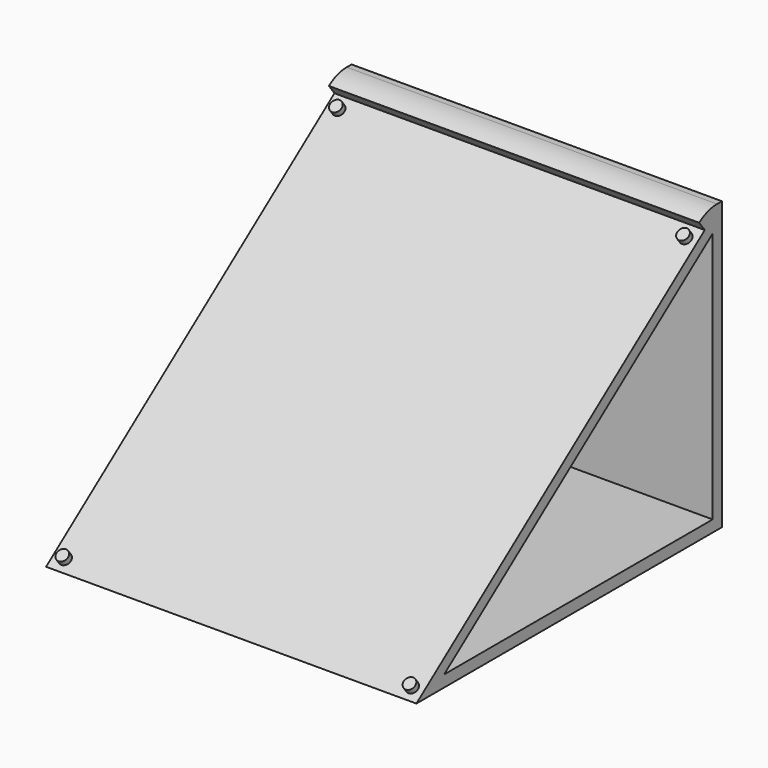
from build123d import *

# Parameters (mm, degrees)
F1_DEPTH  = 50.8
F2_W      = 50.8
F2_H      = 63.5
F2_W_2    = 44.45
F2_H_2    = 57.15
F3_DEPTH  = 1.5875
F5_DEPTH  = 50.8
F6_R      = 5.08
F7_R      = 6.35
F8_DEPTH  = 1.5875
F9_W      = 50.8
F9_H      = 61.8066666667
F9_W_2    = 44.45
F9_H_2    = 57.15
F10_DEPTH = 1.5875
F11_R     = 0.79375
F12_DEPTH = 0.79375
F14_DEPTH = 50.8
F16_DEPTH = 1.5875
F17_T     = -0.79375
F17_2_T   = -0.79375
F17_3_T   = -0.79375
F17_4_T   = -0.79375
F17_5_T   = -0.79375
F17_6_T   = -0.79375
F17_7_T   = -0.79375
F17_8_T   = -0.79375
F17_9_T   = -0.79375
F17_10_T  = -0.79375
F17_11_T  = -0.79375
F17_12_T  = -0.79375
F17_13_T  = -0.79375
F17_14_T  = -0.79375
F17_15_T  = -0.79375
F17_16_T  = -0.79375
F17_17_T  = -0.79375
F17_18_T  = -0.79375
F17_19_T  = -0.79375
F17_20_T  = -0.79375
F17_21_T  = -0.79375
F18_DEPTH = 0.396875


with BuildPart() as f1:
    # F0 (on Right) → F1 (new body)
    with BuildSketch(Plane.YZ):
        Polygon((0, 36.115625), (0, 0), (1.5875, 0), (1.5875, 38.1), (0, 38.1), (-50.8, 0), (-48.1541666667, 0), align=None)
    extrude(amount=F1_DEPTH)

    # F2 (on face) → F3 (join)
    with BuildSketch(Plane(origin=(0, -18.288, 24.384), x_dir=(1, 0, 0), z_dir=(0, -0.6, 0.8))):
        with Locations((25.4, -8.89)):
            Rectangle(F2_W, F2_H)
        with Locations((25.4, -8.89)):
            Rectangle(F2_W_2, F2_H_2, mode=Mode.SUBTRACT)
    extrude(amount=F3_DEPTH)

    # F4 (on face) → F5 (join)
    with BuildSketch(Plane.YZ.offset(50.8)):
        Polygon((0, 38.1), (1.5875, 38.1), (1.5875, 39.37), (-0.9525, 39.37), align=None)
    extrude(amount=-F5_DEPTH)

    # F6
    f6_edges = [f1.edges().sort_by_distance(p)[0] for p in [
        (25.4, -0.9525, 39.37),
    ]]
    fillet(f6_edges, radius=F6_R)

    # F7 (on face) → F8 (cut)
    with BuildSketch(Plane(origin=(0, 1.5875, 0), x_dir=(-1, 0, 0), z_dir=(0, 1, 0))):
        with Locations((-25.4, 19.685)):
            Circle(F7_R)
    extrude(amount=-F8_DEPTH, mode=Mode.SUBTRACT)

    # F9 (on face) → F10 (cut)
    with BuildSketch(Plane(origin=(0, -19.2405, 25.654), x_dir=(1, 0, 0), z_dir=(0, -0.6, 0.8))):
        with Locations((25.4, -9.7366666667)):
            Rectangle(F9_W, F9_H)
        with Locations((25.4, -8.89)):
            Rectangle(F9_W_2, F9_H_2, mode=Mode.SUBTRACT)
    extrude(amount=-F10_DEPTH, mode=Mode.SUBTRACT)

    # F11 (on face) → F12 (join)
    with BuildSketch(Plane(origin=(0, -18.288, 24.384), x_dir=(1, 0, 0), z_dir=(0, -0.6, 0.8))):
        with Locations((1.5875, 19.5791666667)):
            Circle(F11_R)
        with Locations((1.5875, -39.0525)):
            Circle(F11_R)
        with Locations((49.2125, -39.0525)):
            Circle(F11_R)
        with Locations((49.2125, 19.5791666667)):
            Circle(F11_R)
    extrude(amount=F12_DEPTH)

    # F13 (on face) → F14 (join)
    with BuildSketch(Plane.YZ.offset(50.8)):
        Polygon((-46.0375, 1.5875), (-48.1541666667, 0), (0, 0), (0, 1.5875), align=None)
    extrude(amount=-F14_DEPTH)


with BuildPart() as f16:
    # F15 (on face) → F16 (new body)
    with BuildSketch(Plane(origin=(0, 0, 0), x_dir=(0, -1, 0), z_dir=(-1, 0, 0))):
        Polygon((0, 36.115625), (0, 29.765625), (8.4666666667, 29.765625), align=None)
    extrude(amount=-F16_DEPTH)

    # F17
    f17_openings = [f16.faces().sort_by_distance(p)[0] for p in [
        (0, -2.822222, 31.882292),
        (1.5875, -2.822222, 31.882292),
    ]]
    offset(amount=F17_T, openings=f17_openings)


with BuildPart() as f16b:
    # F15 (on face) → F16, piece 2 (new body)
    with BuildSketch(Plane(origin=(0, 0, 0), x_dir=(0, -1, 0), z_dir=(-1, 0, 0))):
        Polygon((8.4666666667, 29.765625), (8.4666666667, 23.415625), (16.9333333333, 23.415625), align=None)
    extrude(amount=-F16_DEPTH)

    # F17#5
    f17_5_openings = [f16b.faces().sort_by_distance(p)[0] for p in [
        (1.5875, -11.288889, 25.532292),
        (0, -11.288889, 25.532292),
    ]]
    offset(amount=F17_5_T, openings=f17_5_openings)


with BuildPart() as f16c:
    # F15 (on face) → F16, piece 3 (new body)
    with BuildSketch(Plane(origin=(0, 0, 0), x_dir=(0, -1, 0), z_dir=(-1, 0, 0))):
        Polygon((16.9333333333, 23.415625), (16.9333333333, 17.065625), (25.4, 17.065625), align=None)
    extrude(amount=-F16_DEPTH)

    # F17#12
    f17_12_openings = [f16c.faces().sort_by_distance(p)[0] for p in [
        (1.5875, -19.755556, 19.182292),
        (0, -19.755556, 19.182292),
    ]]
    offset(amount=F17_12_T, openings=f17_12_openings)


with BuildPart() as f16d:
    # F15 (on face) → F16, piece 4 (new body)
    with BuildSketch(Plane(origin=(0, 0, 0), x_dir=(0, -1, 0), z_dir=(-1, 0, 0))):
        Polygon((25.4, 17.065625), (25.4, 10.715625), (33.8666666667, 10.715625), align=None)
    extrude(amount=-F16_DEPTH)

    # F17#13
    f17_13_openings = [f16d.faces().sort_by_distance(p)[0] for p in [
        (1.5875, -28.222222, 12.832292),
        (0, -28.222222, 12.832292),
    ]]
    offset(amount=F17_13_T, openings=f17_13_openings)


with BuildPart() as f16e:
    # F15 (on face) → F16, piece 5 (new body)
    with BuildSketch(Plane(origin=(0, 0, 0), x_dir=(0, -1, 0), z_dir=(-1, 0, 0))):
        Polygon((33.8666666667, 10.715625), (33.8666666667, 4.365625), (42.3333333333, 4.365625), align=None)
    extrude(amount=-F16_DEPTH)

    # F17#15
    f17_15_openings = [f16e.faces().sort_by_distance(p)[0] for p in [
        (1.5875, -36.688889, 6.482292),
        (0, -36.688889, 6.482292),
    ]]
    offset(amount=F17_15_T, openings=f17_15_openings)


with BuildPart() as f16f:
    # F15 (on face) → F16, piece 6 (new body)
    with BuildSketch(Plane(origin=(0, 0, 0), x_dir=(0, -1, 0), z_dir=(-1, 0, 0))):
        Polygon((46.0375, 1.5875), (42.3333333333, 4.365625), (42.3333333333, 1.5875), align=None)
    extrude(amount=-F16_DEPTH)

    # F17#16
    f17_16_openings = [f16f.faces().sort_by_distance(p)[0] for p in [
        (0, -43.568056, 2.513542),
        (1.5875, -43.568056, 2.513542),
    ]]
    offset(amount=F17_16_T, openings=f17_16_openings)


with BuildPart() as f16g:
    # F15 (on face) → F16, piece 7 (new body)
    with BuildSketch(Plane(origin=(0, 0, 0), x_dir=(0, -1, 0), z_dir=(-1, 0, 0))):
        Polygon((37.5708333333, 1.5875), (33.8666666667, 4.365625), (33.8666666667, 1.5875), align=None)
    extrude(amount=-F16_DEPTH)

    # F17#17
    f17_17_openings = [f16g.faces().sort_by_distance(p)[0] for p in [
        (0, -35.101389, 2.513542),
        (1.5875, -35.101389, 2.513542),
    ]]
    offset(amount=F17_17_T, openings=f17_17_openings)


with BuildPart() as f16h:
    # F15 (on face) → F16, piece 8 (new body)
    with BuildSketch(Plane(origin=(0, 0, 0), x_dir=(0, -1, 0), z_dir=(-1, 0, 0))):
        Polygon((33.8666666667, 4.365625), (25.4, 10.715625), (25.4, 4.365625), align=None)
    extrude(amount=-F16_DEPTH)

    # F17#14
    f17_14_openings = [f16h.faces().sort_by_distance(p)[0] for p in [
        (1.5875, -28.222222, 6.482292),
        (0, -28.222222, 6.482292),
    ]]
    offset(amount=F17_14_T, openings=f17_14_openings)


with BuildPart() as f16i:
    # F15 (on face) → F16, piece 9 (new body)
    with BuildSketch(Plane(origin=(0, 0, 0), x_dir=(0, -1, 0), z_dir=(-1, 0, 0))):
        Polygon((29.1041666667, 1.5875), (25.4, 4.365625), (25.4, 1.5875), align=None)
    extrude(amount=-F16_DEPTH)

    # F17#18
    f17_18_openings = [f16i.faces().sort_by_distance(p)[0] for p in [
        (0, -26.634722, 2.513542),
        (1.5875, -26.634722, 2.513542),
    ]]
    offset(amount=F17_18_T, openings=f17_18_openings)


with BuildPart() as f16j:
    # F15 (on face) → F16, piece 10 (new body)
    with BuildSketch(Plane(origin=(0, 0, 0), x_dir=(0, -1, 0), z_dir=(-1, 0, 0))):
        Polygon((20.6375, 1.5875), (16.9333333333, 4.365625), (16.9333333333, 1.5875), align=None)
    extrude(amount=-F16_DEPTH)

    # F17#19
    f17_19_openings = [f16j.faces().sort_by_distance(p)[0] for p in [
        (0, -18.168056, 2.513542),
        (1.5875, -18.168056, 2.513542),
    ]]
    offset(amount=F17_19_T, openings=f17_19_openings)


with BuildPart() as f16k:
    # F15 (on face) → F16, piece 11 (new body)
    with BuildSketch(Plane(origin=(0, 0, 0), x_dir=(0, -1, 0), z_dir=(-1, 0, 0))):
        Polygon((12.1708333333, 1.5875), (8.4666666667, 4.365625), (8.4666666667, 1.5875), align=None)
    extrude(amount=-F16_DEPTH)

    # F17#20
    f17_20_openings = [f16k.faces().sort_by_distance(p)[0] for p in [
        (0, -9.701389, 2.513542),
        (1.5875, -9.701389, 2.513542),
    ]]
    offset(amount=F17_20_T, openings=f17_20_openings)


with BuildPart() as f16l:
    # F15 (on face) → F16, piece 12 (new body)
    with BuildSketch(Plane(origin=(0, 0, 0), x_dir=(0, -1, 0), z_dir=(-1, 0, 0))):
        Polygon((3.7041666667, 1.5875), (0, 4.365625), (0, 1.5875), align=None)
    extrude(amount=-F16_DEPTH)

    # F17#21
    f17_21_openings = [f16l.faces().sort_by_distance(p)[0] for p in [
        (0, -1.234722, 2.513542),
        (1.5875, -1.234722, 2.513542),
    ]]
    offset(amount=F17_21_T, openings=f17_21_openings)


with BuildPart() as f16m:
    # F15 (on face) → F16, piece 13 (new body)
    with BuildSketch(Plane(origin=(0, 0, 0), x_dir=(0, -1, 0), z_dir=(-1, 0, 0))):
        Polygon((8.4666666667, 4.365625), (0, 10.715625), (0, 4.365625), align=None)
    extrude(amount=-F16_DEPTH)

    # F17#10
    f17_10_openings = [f16m.faces().sort_by_distance(p)[0] for p in [
        (1.5875, -2.822222, 6.482292),
        (0, -2.822222, 6.482292),
    ]]
    offset(amount=F17_10_T, openings=f17_10_openings)


with BuildPart() as f16n:
    # F15 (on face) → F16, piece 14 (new body)
    with BuildSketch(Plane(origin=(0, 0, 0), x_dir=(0, -1, 0), z_dir=(-1, 0, 0))):
        Polygon((8.4666666667, 10.715625), (0, 17.065625), (0, 10.715625), align=None)
    extrude(amount=-F16_DEPTH)

    # F17#6
    f17_6_openings = [f16n.faces().sort_by_distance(p)[0] for p in [
        (1.5875, -2.822222, 12.832292),
        (0, -2.822222, 12.832292),
    ]]
    offset(amount=F17_6_T, openings=f17_6_openings)


with BuildPart() as f16o:
    # F15 (on face) → F16, piece 15 (new body)
    with BuildSketch(Plane(origin=(0, 0, 0), x_dir=(0, -1, 0), z_dir=(-1, 0, 0))):
        Polygon((8.4666666667, 17.065625), (0, 23.415625), (0, 17.065625), align=None)
    extrude(amount=-F16_DEPTH)

    # F17#3
    f17_3_openings = [f16o.faces().sort_by_distance(p)[0] for p in [
        (1.5875, -2.822222, 19.182292),
        (0, -2.822222, 19.182292),
    ]]
    offset(amount=F17_3_T, openings=f17_3_openings)


with BuildPart() as f16p:
    # F15 (on face) → F16, piece 16 (new body)
    with BuildSketch(Plane(origin=(0, 0, 0), x_dir=(0, -1, 0), z_dir=(-1, 0, 0))):
        Polygon((8.4666666667, 23.415625), (0, 29.765625), (0, 23.415625), align=None)
    extrude(amount=-F16_DEPTH)

    # F17#2
    f17_2_openings = [f16p.faces().sort_by_distance(p)[0] for p in [
        (0, -2.822222, 25.532292),
        (1.5875, -2.822222, 25.532292),
    ]]
    offset(amount=F17_2_T, openings=f17_2_openings)


with BuildPart() as f16q:
    # F15 (on face) → F16, piece 17 (new body)
    with BuildSketch(Plane(origin=(0, 0, 0), x_dir=(0, -1, 0), z_dir=(-1, 0, 0))):
        Polygon((16.9333333333, 17.065625), (8.4666666667, 23.415625), (8.4666666667, 17.065625), align=None)
    extrude(amount=-F16_DEPTH)

    # F17#4
    f17_4_openings = [f16q.faces().sort_by_distance(p)[0] for p in [
        (1.5875, -11.288889, 19.182292),
        (0, -11.288889, 19.182292),
    ]]
    offset(amount=F17_4_T, openings=f17_4_openings)


with BuildPart() as f16r:
    # F15 (on face) → F16, piece 18 (new body)
    with BuildSketch(Plane(origin=(0, 0, 0), x_dir=(0, -1, 0), z_dir=(-1, 0, 0))):
        Polygon((16.9333333333, 10.715625), (8.4666666667, 17.065625), (8.4666666667, 10.715625), align=None)
    extrude(amount=-F16_DEPTH)

    # F17#7
    f17_7_openings = [f16r.faces().sort_by_distance(p)[0] for p in [
        (1.5875, -11.288889, 12.832292),
        (0, -11.288889, 12.832292),
    ]]
    offset(amount=F17_7_T, openings=f17_7_openings)


with BuildPart() as f16s:
    # F15 (on face) → F16, piece 19 (new body)
    with BuildSketch(Plane(origin=(0, 0, 0), x_dir=(0, -1, 0), z_dir=(-1, 0, 0))):
        Polygon((16.9333333333, 4.365625), (8.4666666667, 10.715625), (8.4666666667, 4.365625), align=None)
    extrude(amount=-F16_DEPTH)

    # F17#9
    f17_9_openings = [f16s.faces().sort_by_distance(p)[0] for p in [
        (1.5875, -11.288889, 6.482292),
        (0, -11.288889, 6.482292),
    ]]
    offset(amount=F17_9_T, openings=f17_9_openings)


with BuildPart() as f16t:
    # F15 (on face) → F16, piece 20 (new body)
    with BuildSketch(Plane(origin=(0, 0, 0), x_dir=(0, -1, 0), z_dir=(-1, 0, 0))):
        Polygon((25.4, 10.715625), (16.9333333333, 17.065625), (16.9333333333, 10.715625), align=None)
    extrude(amount=-F16_DEPTH)

    # F17#8
    f17_8_openings = [f16t.faces().sort_by_distance(p)[0] for p in [
        (1.5875, -19.755556, 12.832292),
        (0, -19.755556, 12.832292),
    ]]
    offset(amount=F17_8_T, openings=f17_8_openings)


with BuildPart() as f16u:
    # F15 (on face) → F16, piece 21 (new body)
    with BuildSketch(Plane(origin=(0, 0, 0), x_dir=(0, -1, 0), z_dir=(-1, 0, 0))):
        Polygon((25.4, 4.365625), (16.9333333333, 10.715625), (16.9333333333, 4.365625), align=None)
    extrude(amount=-F16_DEPTH)

    # F17#11
    f17_11_openings = [f16u.faces().sort_by_distance(p)[0] for p in [
        (1.5875, -19.755556, 6.482292),
        (0, -19.755556, 6.482292),
    ]]
    offset(amount=F17_11_T, openings=f17_11_openings)


with BuildPart() as f18:
    # F15 (on face) → F18 (new body)
    with BuildSketch(Plane(origin=(0, 0, 0), x_dir=(0, -1, 0), z_dir=(-1, 0, 0))):
        Polygon((8.4666666667, 29.765625), (0, 29.765625), (8.4666666667, 23.415625), align=None)
    extrude(amount=F18_DEPTH)


with BuildPart() as f18b:
    # F15 (on face) → F18, piece 2 (new body)
    with BuildSketch(Plane(origin=(0, 0, 0), x_dir=(0, -1, 0), z_dir=(-1, 0, 0))):
        Polygon((8.4666666667, 17.065625), (8.4666666667, 23.415625), (0, 23.415625), align=None)
    extrude(amount=F18_DEPTH)


with BuildPart() as f18c:
    # F15 (on face) → F18, piece 3 (new body)
    with BuildSketch(Plane(origin=(0, 0, 0), x_dir=(0, -1, 0), z_dir=(-1, 0, 0))):
        Polygon((8.4666666667, 10.715625), (8.4666666667, 17.065625), (0, 17.065625), align=None)
    extrude(amount=F18_DEPTH)


with BuildPart() as f18d:
    # F15 (on face) → F18, piece 4 (new body)
    with BuildSketch(Plane(origin=(0, 0, 0), x_dir=(0, -1, 0), z_dir=(-1, 0, 0))):
        Polygon((8.4666666667, 4.365625), (8.4666666667, 10.715625), (0, 10.715625), align=None)
    extrude(amount=F18_DEPTH)


with BuildPart() as f18e:
    # F15 (on face) → F18, piece 5 (new body)
    with BuildSketch(Plane(origin=(0, 0, 0), x_dir=(0, -1, 0), z_dir=(-1, 0, 0))):
        Polygon((8.4666666667, 1.5875), (8.4666666667, 4.365625), (0, 4.365625), (3.7041666667, 1.5875), align=None)
    extrude(amount=F18_DEPTH)


with BuildPart() as f18f:
    # F15 (on face) → F18, piece 6 (new body)
    with BuildSketch(Plane(origin=(0, 0, 0), x_dir=(0, -1, 0), z_dir=(-1, 0, 0))):
        Polygon((16.9333333333, 1.5875), (16.9333333333, 4.365625), (8.4666666667, 4.365625), (12.1708333333, 1.5875), align=None)
    extrude(amount=F18_DEPTH)


with BuildPart() as f18g:
    # F15 (on face) → F18, piece 7 (new body)
    with BuildSketch(Plane(origin=(0, 0, 0), x_dir=(0, -1, 0), z_dir=(-1, 0, 0))):
        Polygon((25.4, 1.5875), (25.4, 4.365625), (16.9333333333, 4.365625), (20.6375, 1.5875), align=None)
    extrude(amount=F18_DEPTH)


with BuildPart() as f18h:
    # F15 (on face) → F18, piece 8 (new body)
    with BuildSketch(Plane(origin=(0, 0, 0), x_dir=(0, -1, 0), z_dir=(-1, 0, 0))):
        Polygon((33.8666666667, 1.5875), (33.8666666667, 4.365625), (25.4, 4.365625), (29.1041666667, 1.5875), align=None)
    extrude(amount=F18_DEPTH)


with BuildPart() as f18i:
    # F15 (on face) → F18, piece 9 (new body)
    with BuildSketch(Plane(origin=(0, 0, 0), x_dir=(0, -1, 0), z_dir=(-1, 0, 0))):
        Polygon((16.9333333333, 10.715625), (16.9333333333, 17.065625), (8.4666666667, 17.065625), align=None)
    extrude(amount=F18_DEPTH)


with BuildPart() as f18j:
    # F15 (on face) → F18, piece 10 (new body)
    with BuildSketch(Plane(origin=(0, 0, 0), x_dir=(0, -1, 0), z_dir=(-1, 0, 0))):
        Polygon((16.9333333333, 4.365625), (16.9333333333, 10.715625), (8.4666666667, 10.715625), align=None)
    extrude(amount=F18_DEPTH)


with BuildPart() as f18k:
    # F15 (on face) → F18, piece 11 (new body)
    with BuildSketch(Plane(origin=(0, 0, 0), x_dir=(0, -1, 0), z_dir=(-1, 0, 0))):
        Polygon((16.9333333333, 23.415625), (8.4666666667, 23.415625), (16.9333333333, 17.065625), align=None)
    extrude(amount=F18_DEPTH)


with BuildPart() as f18l:
    # F15 (on face) → F18, piece 12 (new body)
    with BuildSketch(Plane(origin=(0, 0, 0), x_dir=(0, -1, 0), z_dir=(-1, 0, 0))):
        Polygon((25.4, 17.065625), (16.9333333333, 17.065625), (25.4, 10.715625), align=None)
    extrude(amount=F18_DEPTH)


with BuildPart() as f18m:
    # F15 (on face) → F18, piece 13 (new body)
    with BuildSketch(Plane(origin=(0, 0, 0), x_dir=(0, -1, 0), z_dir=(-1, 0, 0))):
        Polygon((25.4, 4.365625), (25.4, 10.715625), (16.9333333333, 10.715625), align=None)
    extrude(amount=F18_DEPTH)


with BuildPart() as f18n:
    # F15 (on face) → F18, piece 14 (new body)
    with BuildSketch(Plane(origin=(0, 0, 0), x_dir=(0, -1, 0), z_dir=(-1, 0, 0))):
        Polygon((33.8666666667, 10.715625), (25.4, 10.715625), (33.8666666667, 4.365625), align=None)
    extrude(amount=F18_DEPTH)


with BuildPart() as f18o:
    # F15 (on face) → F18, piece 15 (new body)
    with BuildSketch(Plane(origin=(0, 0, 0), x_dir=(0, -1, 0), z_dir=(-1, 0, 0))):
        Polygon((42.3333333333, 4.365625), (33.8666666667, 4.365625), (37.5708333333, 1.5875), (42.3333333333, 1.5875), align=None)
    extrude(amount=F18_DEPTH)


solid = Compound([f1.part, f16.part, f16b.part, f16c.part, f16d.part, f16e.part, f16f.part, f16g.part, f16h.part, f16i.part, f16j.part, f16k.part, f16l.part, f16m.part, f16n.part, f16o.part, f16p.part, f16q.part, f16r.part, f16s.part, f16t.part, f16u.part, f18.part, f18b.part, f18c.part, f18d.part, f18e.part, f18f.part, f18g.part, f18h.part, f18i.part, f18j.part, f18k.part, f18l.part, f18m.part, f18n.part, f18o.part])
